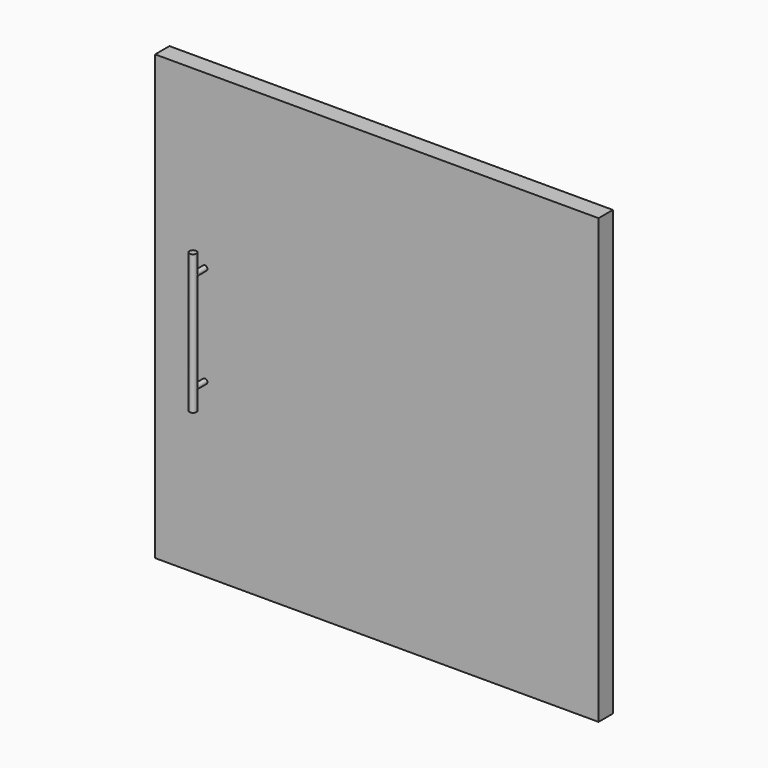
from build123d import *

# Parameters (mm, degrees)
F0_W     = 445
F0_H     = 445
F1_DEPTH = 18
F2_R     = 2.5
F3_DEPTH = 15
F4_R     = 3.5
F5_DEPTH = 70


# Not quite as in the source:
# - a pattern or mirror of a feature is missing from the dataset's text; its kind, count and spacing are read off the source's solid


with BuildPart() as f1:
    # F0 (on Front) → F1 (new body)
    with BuildSketch(Plane.XZ):
        Rectangle(F0_W, F0_H)
    extrude(amount=F1_DEPTH)

    # F2 (on face) → F3 (join)
    with BuildSketch(Plane.XZ.offset(18)):
        with Locations((-172.5, 50)):
            Circle(F2_R)
    f3 = extrude(amount=F3_DEPTH)

    # F3_copies: F3 across plane
    add(f3.mirror(Plane(origin=(0, 0, -1e-05), x_dir=(-1, 0, 0), z_dir=(0, 0, -1))))

    # F4 (on Top) → F5 (join, symmetric)
    with BuildSketch(Plane.XY):
        with Locations((-172.5, -33)):
            Circle(F4_R)
    extrude(amount=F5_DEPTH, both=True)


solid = f1.part
